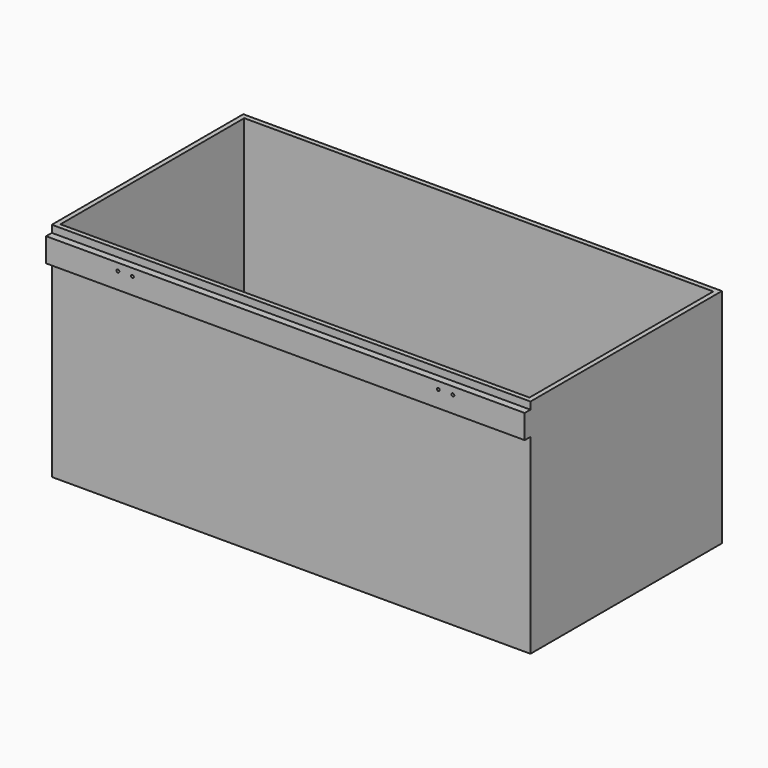
from build123d import *

# Parameters (mm, degrees)
F0_W     = 1000
F0_H     = 500
F1_DEPTH = 464
F2_W     = 980
F2_H     = 480
F3_DEPTH = 10
F4_T     = -10
F5_W     = 1000
F5_H     = 50
F6_DEPTH = 15
F8_D     = 6
F8_DEPTH = 15
F8_TIP   = 1.8025818571


# Not quite as in the source:
# - a shell that OpenCascade refuses in one call is made with other operations: the cavity is built on its own and cut out


with BuildPart() as f1:
    # F0 (on Top) → F1 (new body)
    with BuildSketch(Plane.XY):
        Rectangle(F0_W, F0_H)
    extrude(amount=F1_DEPTH)

    # F2 (on face) → F3 (cut)
    with BuildSketch(Plane(origin=(0, 0, 0), x_dir=(1, 0, 0), z_dir=(0, 0, -1))):
        Rectangle(F2_W, F2_H)
    extrude(amount=-F3_DEPTH, mode=Mode.SUBTRACT)

    # F4: a shell. OpenCascade refuses it in one call, so the cavity is built on its own and cut out:
    # the body offset inwards by the wall thickness, plus a prism from it out through each open face.
    f4_core = offset(f1.part, amount=F4_T, kind=Kind.INTERSECTION, mode=Mode.PRIVATE)
    f4_exits = [f4_core.faces().sort_by_distance(p)[0] for p in [
        (0, 0, 454),
    ]]
    add(f4_core, mode=Mode.SUBTRACT)
    extrude(f4_exits, amount=-F4_T, mode=Mode.SUBTRACT)

    # F5 (on face) → F6 (join)
    with BuildSketch(Plane.XZ.offset(250)):
        with Locations((0, 424)):
            Rectangle(F5_W, F5_H)
    extrude(amount=F6_DEPTH)

    # F8
    with Locations(Plane.XZ.offset(265)):
        with Locations((-350, 433.5), (-319.5, 433.5), (319.5, 433.5), (350, 433.5)):
            Hole(F8_D / 2, depth=F8_DEPTH)
            with Locations((0, 0, -(F8_DEPTH + F8_TIP / 2))):  # 118° drill point
                Cone(0, F8_D / 2, F8_TIP, mode=Mode.SUBTRACT)


solid = f1.part
